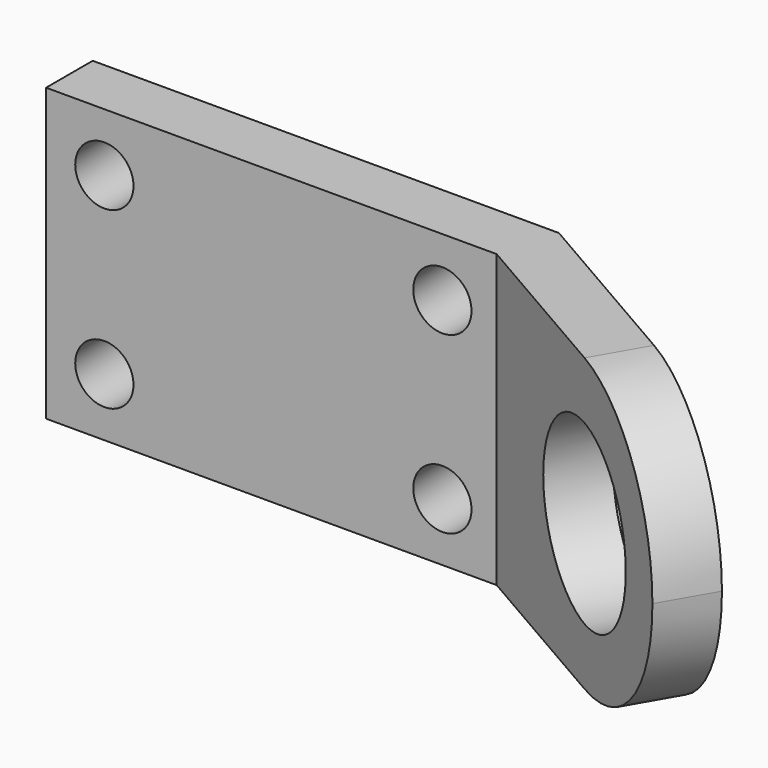
from build123d import *

# Parameters (mm, degrees)
F1_DEPTH = 50
F2_R     = 24.99999
F3_R     = 15.1938434026
F4_DEPTH = 73.4817621135
F5_R     = 5
F6_DEPTH = 38.6612540378


# Not quite as in the source:
# - a fillet or chamfer is up to 0.001 mm smaller than in the source, because OpenCascade refuses the exact size


with BuildPart() as f1:
    # F0 (on Top) → F1 (new body)
    with BuildSketch(Plane.XY):
        Polygon((0, 29.6784242139), (-80, 29.6784242139), (-80, 19.6784242139), (-2.6794919243, 19.6784242139), (46.9615242271, -8.9818298239), (51.9615242271, -0.3215757861), align=None)
    extrude(amount=F1_DEPTH)

    # F2 (radius 25 in the source; OpenCascade refuses exactly that, so slightly less here)
    f2_edges = [f1.edges().sort_by_distance(p)[0] for p in [
        (49.461524, -4.651703, 50),
        (49.461524, -4.651703, 0),
    ]]
    fillet(f2_edges, radius=F2_R)

    # F3 (on face) → F4 (cut, through all)
    with BuildSketch(Plane(origin=(12.8511346568, 22.2588181604, 0), x_dir=(-0.8660254038, 0.5, 0), z_dir=(0.5, 0.8660254038, 0))):
        with Locations((-20.160787893, 25)):
            Circle(F3_R)
    extrude(amount=-F4_DEPTH, mode=Mode.SUBTRACT)

    # F5 (on face) → F6 (cut, through all)
    with BuildSketch(Plane(origin=(0, 29.6784242139, 0), x_dir=(-1, 0, 0), z_dir=(0, 1, 0))):
        with Locations((12, 40)):
            Circle(F5_R)
        with Locations((70, 40)):
            Circle(F5_R)
        with Locations((12, 10)):
            Circle(F5_R)
        with Locations((70, 10)):
            Circle(F5_R)
    extrude(amount=-F6_DEPTH, mode=Mode.SUBTRACT)


solid = f1.part
